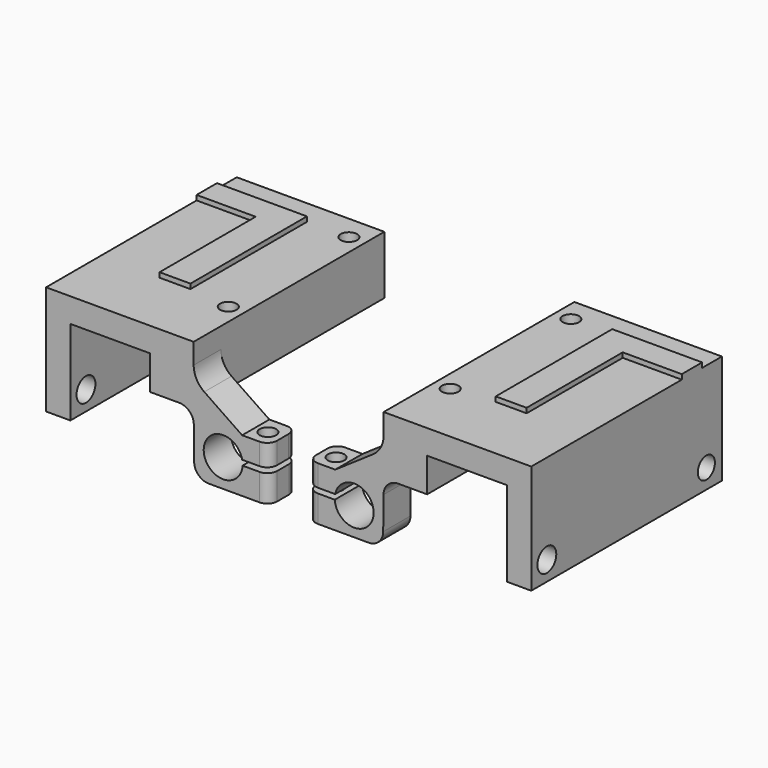
from build123d import *

# Parameters (mm, degrees)
F1_DEPTH      = 7
F2_DEPTH      = 42
F3_R          = 1.7
F3_R_2        = 11
F4_DEPTH      = 12.001
F5_R          = 4
F6_DEPTH      = 10
F7_DEPTH      = 12.001
F8_R          = 1.4
F9_DEPTH      = 10.9920075553
F8_R_2        = 1.7
F10_DEPTH     = 4.4348209087
F11_R         = 5
F12_R         = 3
F13_R         = 3
F14_R         = 2
F15_R         = 2.2
F15_R_2       = 2.4255023423
F16_DEPTH     = 6
F17_TEXT_SIZE = 41.9437823343
F18_DEPTH     = 1


# Not quite as in the source:
# - a feature names something its author has since deleted; it is built from what else it names
# - Text() gives the source's letters only with a copy of the font that has no kerning and outlines rounded to 1/6400 em; it was checked with that copy


with BuildPart() as f1:
    # F0 (on Front) → F1 (new body)
    with BuildSketch(Plane.XZ):
        Polygon((-24.8821007523, 29.8099789735), (-24.8821007523, 7.3259699669), (-19.8821007523, 7.3259699669), (-19.8821007523, 24.8099789735), (-3.4721007523, 24.8099789735), (-3.4721007523, 17.8099789735), (5.4637966118, 17.8099789735), (5.4637966118, 22.9406704692), (5.4637966118, 29.8099789735), align=None)
        Polygon((15.4301751077, 16.1394868046), (5.4637966118, 22.9406704692), (5.4637966118, 17.8099789735), (5.5940201178, 5.1484792493), (21.0186601057, 5.1484792493), (21.0186601057, 10.6682249423), (13.6860510706, 10.6682249423), (13.6860510706, 11.7046658959), (20.9896428882, 11.7046658959), (20.9896428882, 16.1394868046), align=None)
    extrude(amount=F1_DEPTH)

    # F0 (on Front) → F2 (join)
    with BuildSketch(Plane.XZ):
        Polygon((-24.8821007523, 29.8099789735), (-24.8821007523, 7.3259699669), (-19.8821007523, 7.3259699669), (-19.8821007523, 24.8099789735), (-3.4721007523, 24.8099789735), (-3.4721007523, 17.8099789735), (5.4637966118, 17.8099789735), (5.4637966118, 22.9406704692), (5.4637966118, 29.8099789735), align=None)
    extrude(amount=-F2_DEPTH)

    # F3 (on face) → F4 (cut, through all)
    with BuildSketch(Plane(origin=(0, 0, 17.8099789735), x_dir=(1, 0, 0), z_dir=(0, 0, -1))):
        with Locations((2.1850741468, -6)):
            Circle(F3_R)
        with Locations((2.1850741468, -37)):
            Circle(F3_R)
        with Locations((17.6850741468, -21.5)):
            Circle(F3_R_2)
    extrude(amount=-F4_DEPTH, mode=Mode.SUBTRACT)

    # F5 (on face) → F6 (cut)
    with BuildSketch(Plane.XZ.offset(7)):
        with Locations((11.5278992477, 10.8989789735)):
            Circle(F5_R)
    extrude(amount=-F6_DEPTH, mode=Mode.SUBTRACT)

    # F3 (on face) → F7 (cut, through all)
    with BuildSketch(Plane(origin=(0, 0, 17.8099789735), x_dir=(1, 0, 0), z_dir=(0, 0, -1))):
        with Locations((2.1850741468, -6)):
            Circle(F3_R)
        with Locations((2.1850741468, -37)):
            Circle(F3_R)
        with Locations((17.6850741468, -21.5)):
            Circle(F3_R_2)
    extrude(amount=-F7_DEPTH, mode=Mode.SUBTRACT)

    # F8 (on face) → F9 (cut, through all)
    with BuildSketch(Plane.XY.offset(16.1394868046)):
        with Locations((17.9896428882, -3.5767070949)):
            Circle(F8_R)
    extrude(amount=-F9_DEPTH, mode=Mode.SUBTRACT)

    # F8 (on face) → F10 (cut, through all)
    with BuildSketch(Plane.XY.offset(16.1394868046)):
        with Locations((17.9896428882, -3.5767070949)):
            Circle(F8_R_2)
        with Locations((17.9896428882, -3.5767070949)):
            Circle(F8_R, mode=Mode.SUBTRACT)
    extrude(amount=-F10_DEPTH, mode=Mode.SUBTRACT)

    # F11
    f11_edges = [f1.edges().sort_by_distance(p)[0] for p in [
        (5.463797, -3.5, 22.94067),
    ]]
    fillet(f11_edges, radius=F11_R)

    # F12
    f12_edges = [f1.edges().sort_by_distance(p)[0] for p in [
        (5.463797, -3.5, 17.809979),
    ]]
    fillet(f12_edges, radius=F12_R)

    # F13
    f13_edges = [f1.edges().sort_by_distance(p)[0] for p in [
        (5.59402, -3.5, 5.148479),
    ]]
    fillet(f13_edges, radius=F13_R)

    # F14
    f14_edges = [f1.edges().sort_by_distance(p)[0] for p in [
        (20.989643, -7, 13.922076),
        (21.01866, -7, 7.908352),
        (20.989643, 0, 13.922076),
        (21.01866, 0, 7.908352),
    ]]
    fillet(f14_edges, radius=F14_R)

    # F15 (on face) → F16 (cut)
    with BuildSketch(Plane(origin=(-24.8821007523, 0, 0), x_dir=(0, -1, 0), z_dir=(-1, 0, 0))):
        with Locations((-38, 11.3259699669)):
            Circle(F15_R)
        with Locations((3, 11.3259699669)):
            Circle(F15_R_2)
    extrude(amount=-F16_DEPTH, mode=Mode.SUBTRACT)

    # F17 (on face) → F18 (join)
    with BuildSketch(Plane.XY.offset(29.8099789735)):
        with Locations(Location((-2.6191275352, 36.9253193088), (0, 0, 180))):
            Text('L', F17_TEXT_SIZE, font='Open Sans', font_style=FontStyle.BOLD, text_align=(TextAlign.LEFT, TextAlign.BOTTOM))
    extrude(amount=F18_DEPTH)


with BuildPart() as f19_1:
    # F19: instance of F1
    add(f1.part.mirror(Plane.YZ))


with BuildPart() as f19_1_1:
    # F20: moved
    add(f19_1.part.moved(Location((50, 0, 0))))


solid = Compound([f1.part, f19_1_1.part])
